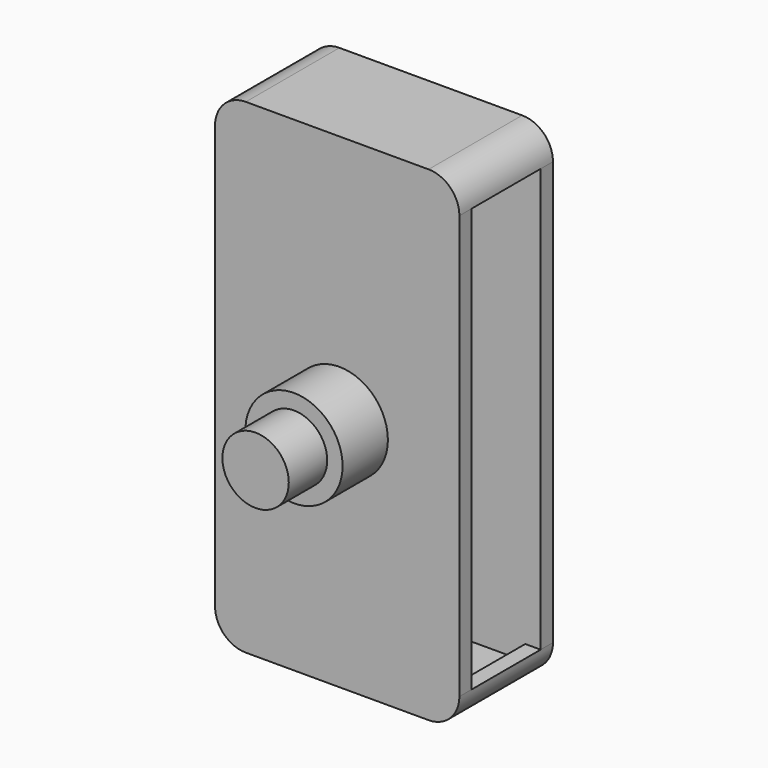
from build123d import *

# Parameters (mm, degrees)
F0_R     = 7.8929339783
F1_DEPTH = 9.2
F2_T     = -2.5
F3_DEPTH = 14.5
F4_W     = 39.6901145577
F4_H     = 78.7652172148
F5_DEPTH = 19
F6_R     = 5
F7_T     = -2.5


# Not quite as in the source:
# - a shell that OpenCascade refuses in one call is made with other operations: the cavity is built on its own and cut out


with BuildPart() as f1:
    # F0 (on Front) → F1 (new body)
    with BuildSketch(Plane.XZ):
        Circle(F0_R)
    extrude(amount=F1_DEPTH)

    # F2
    f2_openings = [f1.faces().sort_by_distance(p)[0] for p in [
        (0, -9.2, 0),
    ]]
    offset(amount=F2_T, openings=f2_openings)

    # F3 (add): a face of the model
    f3_faces = [f1.faces().sort_by_distance(p)[0] for p in [
        (0, -2.5, 0),
    ]]
    extrude(f3_faces, amount=F3_DEPTH)

    # F4 (on Front) → F5 (join)
    with BuildSketch(Plane.XZ):
        with Locations((-0.3387015313, 1.4586504549)):
            Rectangle(F4_W, F4_H)
    extrude(amount=-F5_DEPTH)

    # F6
    f6_edges = [f1.edges().sort_by_distance(p)[0] for p in [
        (19.506356, 9.5, 40.841259),
        (19.506356, 9.5, -37.923958),
        (-20.183759, 9.5, 40.841259),
        (-20.183759, 9.5, -37.923958),
    ]]
    fillet(f6_edges, radius=F6_R)

    # F7: a shell. OpenCascade refuses it in one call, so the cavity is built on its own and cut out:
    # the body offset inwards by the wall thickness, plus a prism from it out through each open face.
    f7_core = offset(f1.part, amount=F7_T, kind=Kind.INTERSECTION, mode=Mode.PRIVATE)
    f7_exits = [f7_core.faces().sort_by_distance(p)[0] for p in [
        (17.006356, 9.5, 1.45865),
        (-17.683759, 9.5, 1.45865),
    ]]
    add(f7_core, mode=Mode.SUBTRACT)
    extrude(f7_exits, amount=-F7_T, mode=Mode.SUBTRACT)


solid = f1.part
